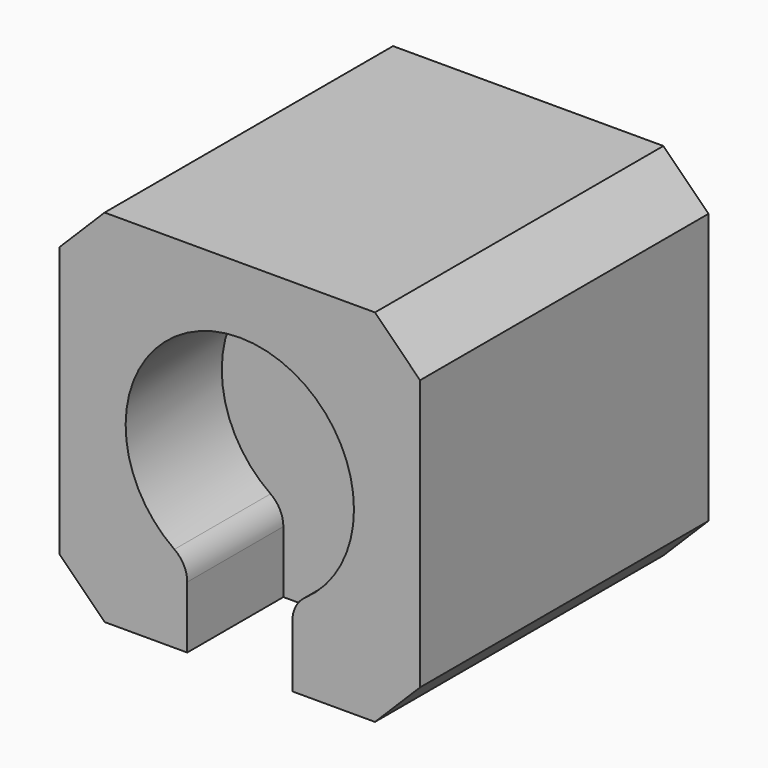
from build123d import *

# Parameters (mm, degrees)
F0_W     = 24
F0_H     = 24
F1_DEPTH = 12
F2_SIZE  = 3
F5_DEPTH = 8
F6_DEPTH = 8
F7_R     = 2


with BuildPart() as f1:
    # F0 (on Front) → F1 (new body, symmetric)
    with BuildSketch(Plane.XZ):
        Rectangle(F0_W, F0_H)
    extrude(amount=F1_DEPTH, both=True)

    # F2
    f2_edges = [f1.edges().sort_by_distance(p)[0] for p in [
        (12, 0, 12),
        (12, 0, -12),
        (-12, 0, -12),
        (-12, 0, 12),
    ]]
    chamfer(f2_edges, length=F2_SIZE)

    # F3 (on face) → F5 (cut)
    with BuildSketch(Plane.XZ.offset(12)):
        with BuildLine():
            ThreePointArc((3.5, -6.7461099902), (6.4946131525, -3.9471508712), (7.6, 0))
            ThreePointArc((7.6, 0), (-3.9471508712, 6.4946131525), (-3.5, -6.7461099902))
            Line((-3.5, -6.7461099902), (-3.5, -5.0646187738))
            Line((-3.5, -5.0646187738), (3.5, -5.0646187738))
            Line((3.5, -5.0646187738), (3.5, -6.7461099902))
        make_face()
        with BuildLine():
            Line((-3.5, -5.0646187738), (-3.5, -6.7461099902))
            ThreePointArc((-3.5, -6.7461099902), (0, -7.6), (3.5, -6.7461099902))
            Line((3.5, -6.7461099902), (3.5, -5.0646187738))
            Line((3.5, -5.0646187738), (-3.5, -5.0646187738))
        make_face()
        with BuildLine():
            ThreePointArc((3.5, -6.7461099902), (0, -7.6), (-3.5, -6.7461099902))
            Line((-3.5, -6.7461099902), (-3.5, -12))
            Line((-3.5, -12), (3.5, -12))
            Line((3.5, -12), (3.5, -6.7461099902))
        make_face()
    extrude(amount=-F5_DEPTH, mode=Mode.SUBTRACT)

    # F4 (on face) → F6 (cut)
    with BuildSketch(Plane(origin=(0, 12, 0), x_dir=(-1, 0, 0), z_dir=(0, 1, 0))):
        with BuildLine():
            ThreePointArc((3.5, -6.7461099902), (6.4946131525, -3.9471508712), (7.6, 0))
            ThreePointArc((7.6, 0), (-3.9471508712, 6.4946131525), (-3.5, -6.7461099902))
            Line((-3.5, -6.7461099902), (-3.5, -5))
            Line((-3.5, -5), (3.5, -5))
            Line((3.5, -5), (3.5, -6.7461099902))
        make_face()
        with BuildLine():
            Line((-3.5, -5), (-3.5, -6.7461099902))
            ThreePointArc((-3.5, -6.7461099902), (0, -7.6), (3.5, -6.7461099902))
            Line((3.5, -6.7461099902), (3.5, -5))
            Line((3.5, -5), (-3.5, -5))
        make_face()
        with BuildLine():
            ThreePointArc((3.5, -6.7461099902), (0, -7.6), (-3.5, -6.7461099902))
            Line((-3.5, -6.7461099902), (-3.5, -12))
            Line((-3.5, -12), (3.5, -12))
            Line((3.5, -12), (3.5, -6.7461099902))
        make_face()
    extrude(amount=-F6_DEPTH, mode=Mode.SUBTRACT)

    # F7
    f7_edges = [f1.edges().sort_by_distance(p)[0] for p in [
        (3.5, 8, -6.74611),
        (-3.5, 8, -6.74611),
        (3.5, -8, -6.74611),
        (-3.5, -8, -6.74611),
    ]]
    fillet(f7_edges, radius=F7_R)


with BuildPart() as f8_1:
    # F8: copy of F1
    add(f1.part)


solid = Compound([f1.part, f8_1.part])
